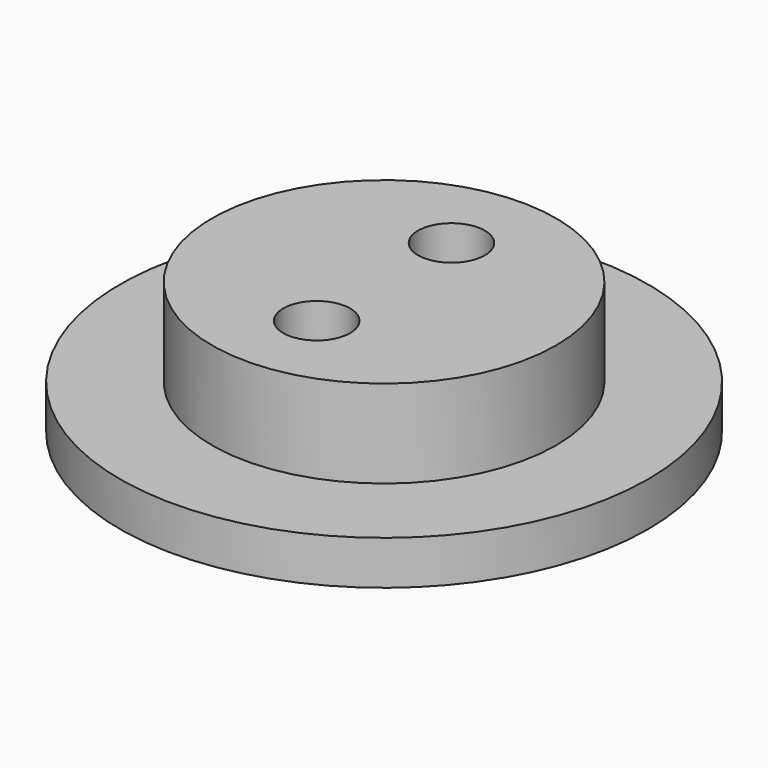
from build123d import *

# Parameters (mm, degrees)
F1_R     = 19.05
F1_R_2   = 2.413
F2_DEPTH = 3.175
F3_R     = 12.4201168804
F3_R_2   = 2.413
F4_DEPTH = 6.35


# Not quite as in the source:
# - a length typed as a fraction of an inch, garbled in the dataset ("3 / 203.2 mm" for 3/8 in), is restored


with BuildPart() as f2:
    # F1 (on Top) → F2 (new body)
    with BuildSketch(Plane.XY):
        with Locations((-45.3916713595, 36.9166433811)):
            Circle(F1_R)
        with Locations((-45.3916713595, 30.8369403438)):
            Circle(F1_R_2, mode=Mode.SUBTRACT)
        with Locations((-45.3916713595, 42.9963464184)):
            Circle(F1_R_2, mode=Mode.SUBTRACT)
    extrude(amount=F2_DEPTH)


with BuildPart() as f4:
    # F3 (on face) → F4 (new body)
    with BuildSketch(Plane.XY.offset(3.175)):
        with Locations((-45.3916713595, 36.9166433811)):
            Circle(F3_R)
        with Locations((-45.3916713595, 30.8369403438)):
            Circle(F3_R_2, mode=Mode.SUBTRACT)
        with Locations((-45.3916713595, 42.9963464184)):
            Circle(F3_R_2, mode=Mode.SUBTRACT)
    extrude(amount=F4_DEPTH)


solid = Compound([f2.part, f4.part])
